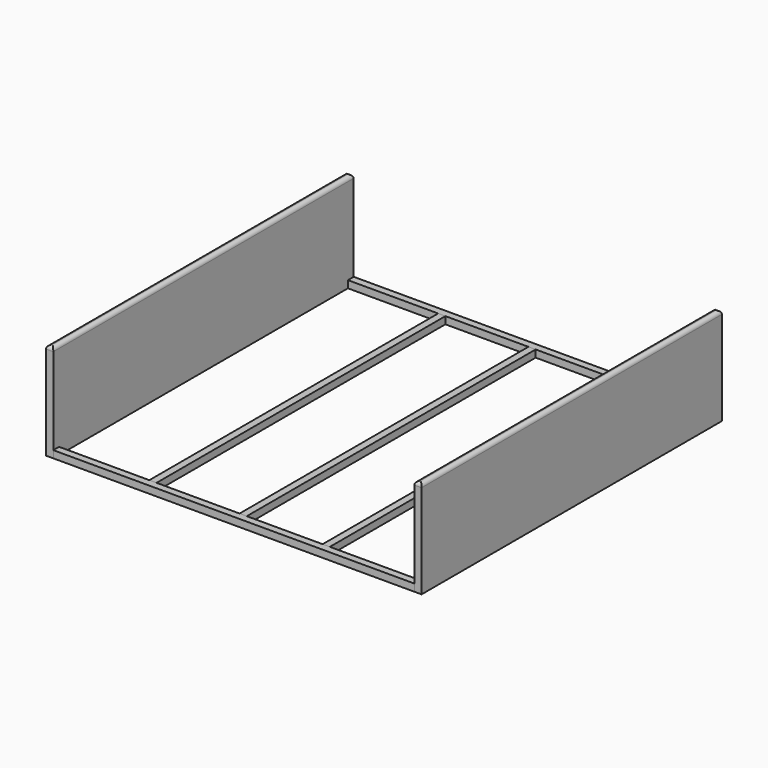
from build123d import *

# Parameters (mm, degrees)
F0_W      = 2
F0_H      = 104
F1_DEPTH  = 27
F2_R      = 0.99999
F4_W      = 2
F4_H      = 104
F5_DEPTH  = 27
F6_R      = 0.99999
F7_W      = 2
F7_H      = 100
F8_DEPTH  = 2
F9_W      = 2
F9_H      = 100
F10_DEPTH = 2
F11_W     = 2
F11_H     = 100
F12_DEPTH = 2
F13_ANGLE = 90
F17_ANGLE = 90


# Not quite as in the source:
# - a fillet or chamfer is up to 0.001 mm smaller than in the source, because OpenCascade refuses the exact size


with BuildPart() as f1:
    # F0 (on Top) → F1 (new body)
    with BuildSketch(Plane.XY):
        with Locations((0, 2)):
            Rectangle(F0_W, F0_H)
    extrude(amount=F1_DEPTH)

    # F2 (radius 1 in the source; OpenCascade refuses exactly that, so slightly less here)
    f2_edges = [f1.edges().sort_by_distance(p)[0] for p in [
        (0, 54, 27),
        (-1, 2, 27),
        (0, -50, 27),
        (1, 2, 27),
    ]]
    fillet(f2_edges, radius=F2_R)


with BuildPart() as f1_1:
    # F3: moved
    add(f1.part.moved(Location((50, 0, 0))))


with BuildPart() as f5:
    # F4 (on Top) → F5 (new body)
    with BuildSketch(Plane.XY):
        with Locations((-52, 2)):
            Rectangle(F4_W, F4_H)
    extrude(amount=F5_DEPTH)

    # F6 (radius 1 in the source; OpenCascade refuses exactly that, so slightly less here)
    f6_edges = [f5.edges().sort_by_distance(p)[0] for p in [
        (-52, 54, 27),
        (-53, 2, 27),
        (-52, -50, 27),
        (-51, 2, 27),
    ]]
    fillet(f6_edges, radius=F6_R)


with BuildPart() as f8:
    # F7 (on Top) → F8 (new body)
    with BuildSketch(Plane.XY):
        with Locations((-25, 0)):
            Rectangle(F7_W, F7_H)
    extrude(amount=F8_DEPTH)


with BuildPart() as f10:
    # F9 (on Top) → F10 (new body)
    with BuildSketch(Plane.XY):
        with Locations((23, 0)):
            Rectangle(F9_W, F9_H)
    extrude(amount=F10_DEPTH)


with BuildPart() as f12:
    # F11 (on Top) → F12 (new body)
    with BuildSketch(Plane.XY):
        Rectangle(F11_W, F11_H)
    extrude(amount=F12_DEPTH)


with BuildPart() as f13_1:
    # F13: copy of F12
    add(f12.part.rotate(Axis((-1, -50, 1), (0, 0, -1)), F13_ANGLE))


with BuildPart() as f13_1_1:
    # F14: moved
    add(f13_1.part.moved(Location((-50, 0, 0))))


with BuildPart() as f5_1:
    # F15: moved
    add(f5.part.moved(Location((0, -2, 0))))


with BuildPart() as f1_2:
    # F16: moved
    add(f1_1.part.moved(Location((0, -2, 0))))


with BuildPart() as f17_1:
    # F17: copy of F12
    add(f12.part.rotate(Axis((-1, 50, 1), (0, 0, -1)), F17_ANGLE))


with BuildPart() as f17_1_1:
    # F18: moved
    add(f17_1.part.moved(Location((0, 2, 0))))


with BuildPart() as f17_1_2:
    # F19: moved
    add(f17_1_1.part.moved(Location((50, 0, 0))))


solid = Compound([f8.part, f10.part, f12.part, f13_1_1.part, f5_1.part, f1_2.part, f17_1_2.part])
